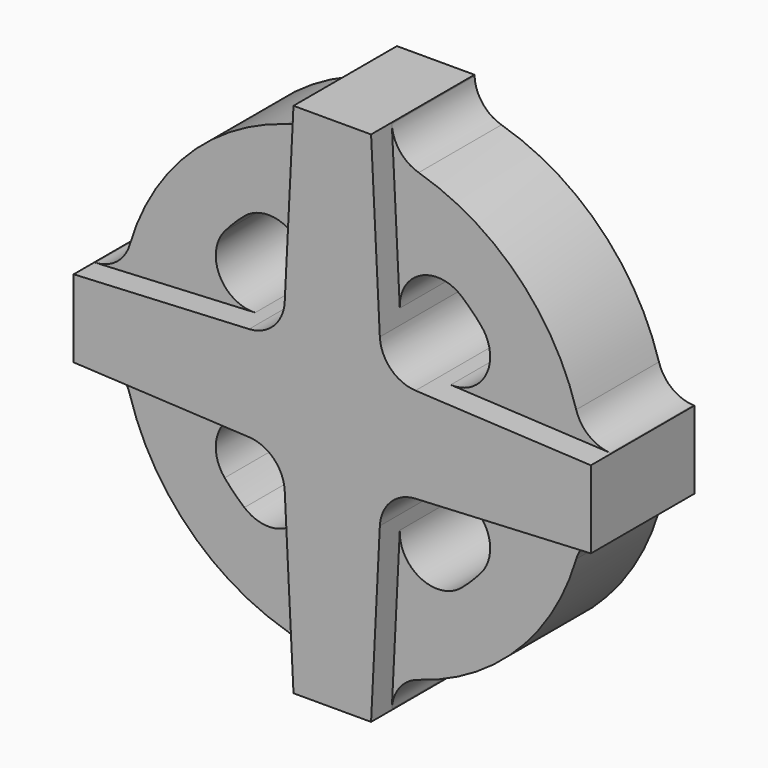
from build123d import *

# Parameters (mm, degrees)
F0_R     = 11.43
F1_DEPTH = 5.08
F3_D     = 16.51
F5_DEPTH = 6.35
F6_R     = 1.84404


# Not quite as in the source:
# - a feature names something its author has since deleted; it is built from what else it names


with BuildPart() as f1:
    # F0 (on Front) → F1 (new body)
    with BuildSketch(Plane.XZ):
        Circle(F0_R)
    extrude(amount=F1_DEPTH)

    # F3 (through all)
    with Locations(Plane.XZ.offset(5.08)):
        with Locations((0, 0)):
            Hole(F3_D / 2)

    # F4 (on Front) → F5 (join)
    with BuildSketch(Plane.XZ):
        Polygon((-2.419047619, -2.419047619), (-2.54, 0), (-2.419047619, 2.419047619), (-12.7, 1.905), (-12.7, -1.905), align=None)
        Polygon((0, -2.54), (-2.419047619, -2.419047619), (-1.905, -12.7), (1.905, -12.7), (2.419047619, -2.419047619), align=None)
        Polygon((2.419047619, 2.419047619), (2.54, 0), (2.419047619, -2.419047619), (12.7, -1.905), (12.7, 1.905), align=None)
        Polygon((-1.905, 12.7), (-2.419047619, 2.419047619), (0, 2.54), (2.419047619, 2.419047619), (1.905, 12.7), align=None)
        Polygon((0, 0), (-2.54, 0), (-2.419047619, -2.419047619), (0, -2.54), align=None)
        Polygon((0, 2.54), (0, 0), (2.54, 0), (2.419047619, 2.419047619), align=None)
        Polygon((-2.419047619, 2.419047619), (-2.54, 0), (0, 0), (0, 2.54), align=None)
        Polygon((2.54, 0), (0, 0), (0, -2.54), (2.419047619, -2.419047619), align=None)
    extrude(amount=F5_DEPTH)

    # F6
    f6_edges = [f1.edges().sort_by_distance(p)[0] for p in [
        (-2.419048, -3.175, -2.419048),
        (-2.419048, -3.175, 2.419048),
        (2.419048, -3.175, 2.419048),
        (2.419048, -3.175, -2.419048),
        (-11.257705, -2.54, -1.977115),
        (-1.977115, -2.54, -11.257705),
        (1.977115, -2.54, -11.257705),
        (11.257705, -2.54, -1.977115),
        (11.257705, -2.54, 1.977115),
        (1.977115, -2.54, 11.257705),
        (-1.977115, -2.54, 11.257705),
        (-11.257705, -2.54, 1.977115),
        (7.972423, -2.54, 2.141379),
        (7.972423, -2.54, -2.141379),
        (2.141379, -2.54, -7.972423),
        (-2.141379, -2.54, -7.972423),
        (-7.972423, -2.54, -2.141379),
        (-7.972423, -2.54, 2.141379),
        (-2.141379, -2.54, 7.972423),
        (2.141379, -2.54, 7.972423),
    ]]
    fillet(f6_edges, radius=F6_R)


solid = f1.part
